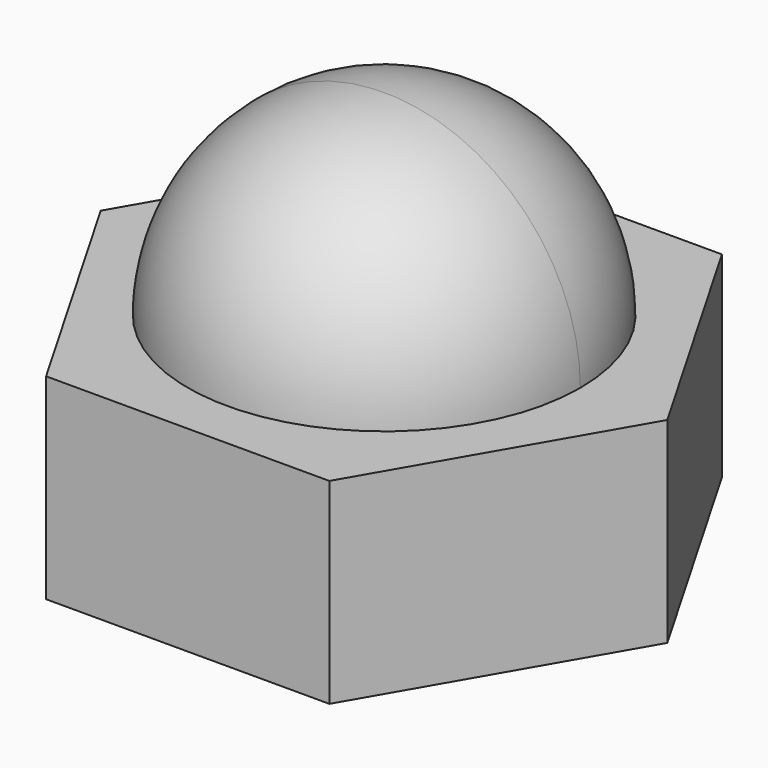
from build123d import *
from build123d import SkipClean  # not in build123d's __all__

# Parameters (mm, degrees)
F1_DEPTH = 4


with BuildPart() as f1:
    # F0 (on Top) → F1 (new body)
    with BuildSketch(Plane.XY):
        Polygon((2.8867513459, 5), (-2.8867513459, 5), (-5.7735026919, 0), (-2.8867513459, -5), (2.8867513459, -5), (5.7735026919, 0), align=None)
    extrude(amount=F1_DEPTH)

    # F2 (on Front) → F3 (revolve)
    with BuildSketch(Plane.XZ):
        with BuildLine():
            Line((-3.9975453725, 4), (4.0024546275, 4))
            ThreePointArc((4.0024546275, 4), (0.0024546275, 8), (-3.9975453725, 4))
        make_face()
    with SkipClean():  # cleaning this boolean's faces spoils the solid; the shape is the same uncleaned
        revolve(axis=Axis((0.0024546275, 0, 4), (1, 0, 0)))


solid = f1.part
